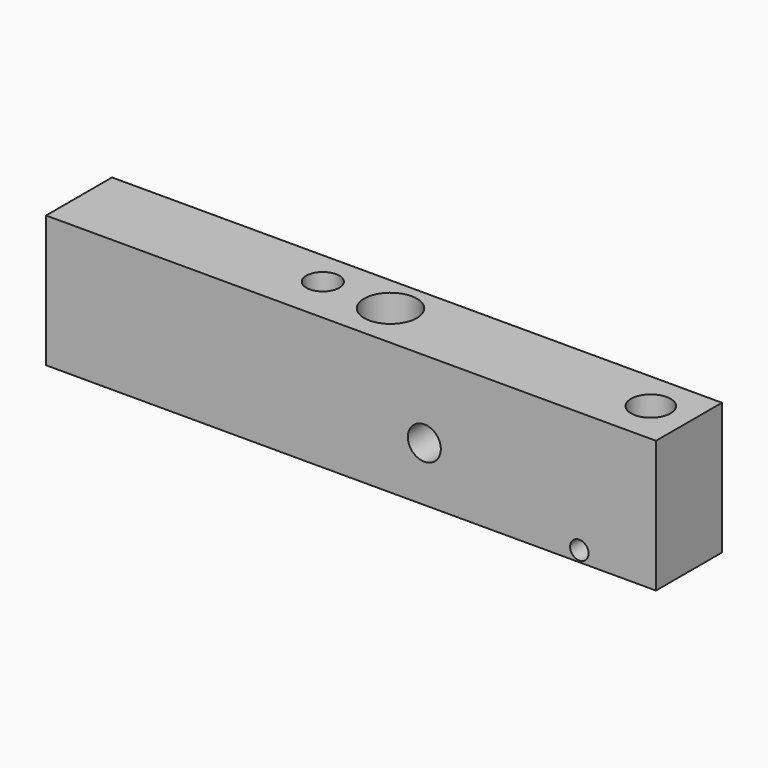
from build123d import *

# Parameters (mm, degrees)
F0_W      = 117.475
F0_H      = 25.4
F1_DEPTH  = 15.875
F3_D      = 6.35
F3_DEPTH  = 177.8
F3_TIP    = 1.9077324654
F5_D      = 10.16
F5_DEPTH  = 177.8
F5_TIP    = 3.0523719447
F7_D      = 7.62
F7_DEPTH  = 177.8
F7_TIP    = 2.2892789585
F9_D      = 6.35
F9_DEPTH  = 177.8
F9_TIP    = 1.9077324654
F11_D     = 3.556
F11_DEPTH = 25.4
F11_TIP   = 1.0683301806


# Not quite as in the source:
# - a feature names something its author has since deleted; it is built from what else it names


with BuildPart() as f1:
    # F0 (on Front) → F1 (new body)
    with BuildSketch(Plane.XZ):
        with Locations((58.7375, 12.7)):
            Rectangle(F0_W, F0_H)
    extrude(amount=F1_DEPTH)

    # F3
    with Locations(Plane(origin=(0, 0, 0), x_dir=(1, 0, 0), z_dir=(0, 0, -1))):
        with Locations((45.984800905, 6.7214882001)):
            Hole(F3_D / 2, depth=F3_DEPTH)
            with Locations((0, 0, -(F3_DEPTH + F3_TIP / 2))):  # 118° drill point
                Cone(0, F3_D / 2, F3_TIP, mode=Mode.SUBTRACT)

    # F5
    with Locations(Plane(origin=(0, 0, 0), x_dir=(1, 0, 0), z_dir=(0, 0, -1))):
        with Locations((59.3467913568, 7.1263969876)):
            Hole(F5_D / 2, depth=F5_DEPTH)
            with Locations((0, 0, -(F5_DEPTH + F5_TIP / 2))):  # 118° drill point
                Cone(0, F5_D / 2, F5_TIP, mode=Mode.SUBTRACT)

    # F7
    with Locations(Plane(origin=(0, 0, 0), x_dir=(1, 0, 0), z_dir=(0, 0, -1))):
        with Locations((109.7984462976, 7.531305775)):
            Hole(F7_D / 2, depth=F7_DEPTH)
            with Locations((0, 0, -(F7_DEPTH + F7_TIP / 2))):  # 118° drill point
                Cone(0, F7_D / 2, F7_TIP, mode=Mode.SUBTRACT)

    # F9
    with Locations(Plane(origin=(0, 0, 0), x_dir=(1, 0, 0), z_dir=(0, 1, 0))):
        with Locations((72.8548616171, -10.5120344087)):
            Hole(F9_D / 2, depth=F9_DEPTH)
            with Locations((0, 0, -(F9_DEPTH + F9_TIP / 2))):  # 118° drill point
                Cone(0, F9_D / 2, F9_TIP, mode=Mode.SUBTRACT)

    # F11
    with Locations(Plane(origin=(0, 0, 0), x_dir=(1, 0, 0), z_dir=(0, 1, 0))):
        with Locations((102.7114540339, -2.0629046485)):
            Hole(F11_D / 2, depth=F11_DEPTH)
            with Locations((0, 0, -(F11_DEPTH + F11_TIP / 2))):  # 118° drill point
                Cone(0, F11_D / 2, F11_TIP, mode=Mode.SUBTRACT)


solid = f1.part
